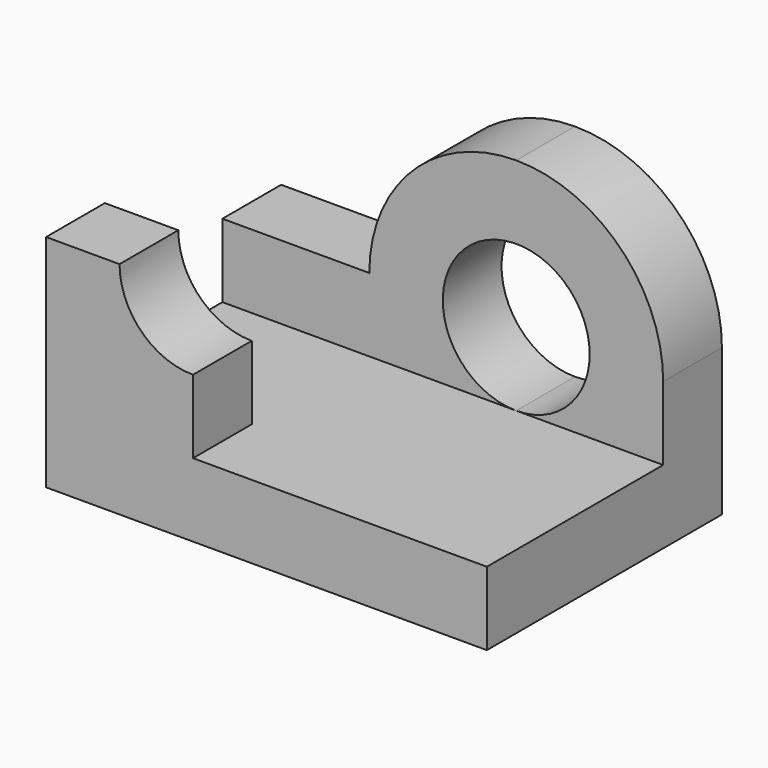
from build123d import *

# Parameters (mm, degrees)
F0_W      = 60
F0_H      = 40
F1_DEPTH  = 10
F2_W      = 60
F2_H      = 10
F3_DEPTH  = 30
F4_W      = 20
F4_H      = 10
F5_DEPTH  = 20
F6_R      = 19.99999
F8_DEPTH  = 10
F9_W      = 20
F9_H      = 10
F10_DEPTH = 20
F12_DEPTH = 10


# Not quite as in the source:
# - a fillet or chamfer is up to 0.001 mm smaller than in the source, because OpenCascade refuses the exact size


with BuildPart() as f1:
    # F0 (on Top) → F1 (new body)
    with BuildSketch(Plane.XY):
        with Locations((-2.2019557655, 9.2856339355)):
            Rectangle(F0_W, F0_H)
    extrude(amount=F1_DEPTH)

    # F2 (on face) → F3 (join)
    with BuildSketch(Plane.XY.offset(10)):
        with Locations((-2.2019557655, 24.2856339355)):
            Rectangle(F2_W, F2_H)
    extrude(amount=F3_DEPTH)

    # F4 (on face) → F5 (cut)
    with BuildSketch(Plane.XY.offset(40)):
        with Locations((-22.2019557655, 24.2856339355)):
            Rectangle(F4_W, F4_H)
    extrude(amount=-F5_DEPTH, mode=Mode.SUBTRACT)

    # F6 (radius 20 in the source; OpenCascade refuses exactly that, so slightly less here)
    f6_edges = [f1.edges().sort_by_distance(p)[0] for p in [
        (-12.201956, 24.285634, 40),
        (27.798044, 24.285634, 40),
    ]]
    fillet(f6_edges, radius=F6_R)

    # F7 (on face) → F8 (cut)
    with BuildSketch(Plane.XZ.offset(-19.2856339355)):
        with BuildLine():
            ThreePointArc((7.7980442039, 10), (14.8691120356, 12.9289321773), (17.7980442345, 20))
            ThreePointArc((17.7980442345, 20), (0.7269764335, 27.0710678227), (7.7980442039, 10))
        make_face()
    extrude(amount=-F8_DEPTH, mode=Mode.SUBTRACT)

    # F9 (on face) → F10 (join)
    with BuildSketch(Plane.XY.offset(10)):
        with Locations((-22.2019557655, -5.7143660645)):
            Rectangle(F9_W, F9_H)
    extrude(amount=F10_DEPTH)

    # F11 (on face) → F12 (cut)
    with BuildSketch(Plane.XZ.offset(10.7143660645)):
        with BuildLine():
            Line((-12.2019557655, 30), (-22.2019557655, 30))
            ThreePointArc((-22.2019557655, 30), (-19.2730235774, 22.9289321881), (-12.2019557655, 20))
            Line((-12.2019557655, 20), (-12.2019557655, 30))
        make_face()
    extrude(amount=-F12_DEPTH, mode=Mode.SUBTRACT)


solid = f1.part
